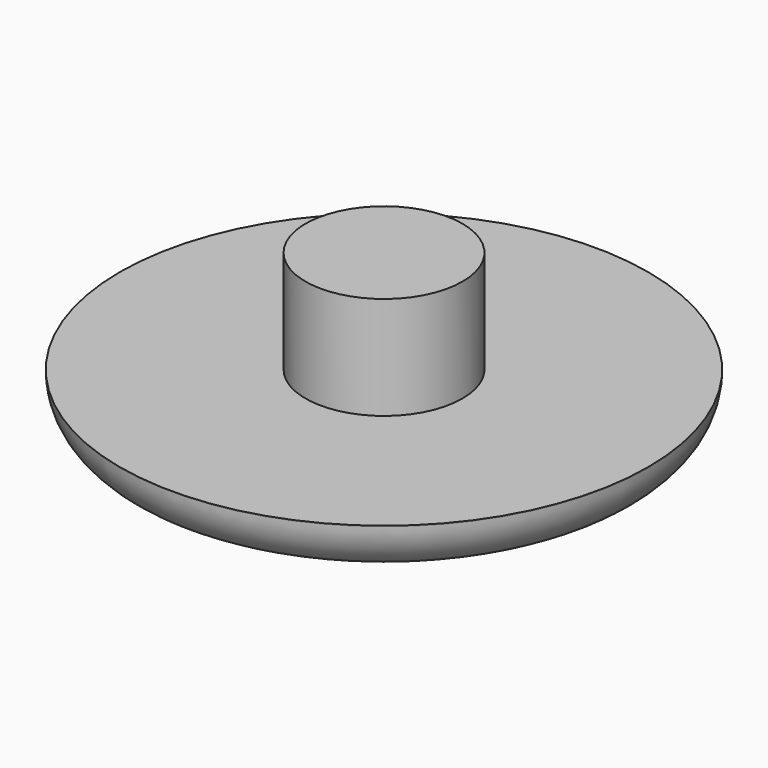
from build123d import *

# Parameters (mm, degrees)
F0_R     = 12.827
F1_DEPTH = 2.54
F2_R     = 8.89
F3_DEPTH = 0.635
F5_R     = 25.4
F7_R     = 3.81
F8_DEPTH = 5


# Not quite as in the source:
# - a fillet or chamfer that OpenCascade refuses, or shapes differently, is made with other operations: its cross-section is extruded or revolved along the edge and cut away or added


with BuildPart() as f1:
    # F0 (on Top) → F1 (new body)
    with BuildSketch(Plane.XY):
        Circle(F0_R)
    extrude(amount=-F1_DEPTH)

    # F2 (on face) → F3 (cut)
    with BuildSketch(Plane(origin=(0, 0, -2.54), x_dir=(1, 0, 0), z_dir=(0, 0, -1))):
        Circle(F2_R)
    extrude(amount=-F3_DEPTH, mode=Mode.SUBTRACT)

    # F4: fillet of radius 60.96 on 1 edges, made by hand

    # F4_s1 → F4_t2 (revolve)
    with BuildSketch(Plane.XZ):
        with BuildLine():
            ThreePointArc((8.89, -2.54), (4.5135344509, -2.0639572458), (0.1141253997, -1.905))
            Line((0.1141253997, -1.905), (8.89, -1.905))
            Line((8.89, -1.905), (8.89, -2.54))
        make_face()
    revolve(axis=Axis((0, 0, -1.905), (0, 0, -1)))

    # F5
    f5_edges = [f1.edges().sort_by_distance(p)[0] for p in [
        (-8.89, 0, -2.54),
    ]]
    fillet(f5_edges, radius=F5_R)

    # F6: fillet of radius 2.54 on 1 edges, made by hand

    # F6_s1 → F6_t2 (revolve, cut)
    with BuildSketch(Plane.XZ):
        with BuildLine():
            ThreePointArc((10.2547372433, -2.5384738057), (12.0719517601, -1.8053490766), (12.8274, 0.0026991598))
            Line((12.8274, 0.0026991598), (13.0815365685, 0.0026991598))
            ThreePointArc((13.0815365685, 0.0026991598), (13.0811365685, -1.2686504201), (13.0811365685, -2.54))
            Line((13.0811365685, -2.54), (12.827, -2.7941365685))
            ThreePointArc((12.827, -2.7941365685), (10.5675446967, -2.7941365685), (10.2516075362, -2.7925911022))
            Line((10.2516075362, -2.7925911022), (10.2547372433, -2.5384738057))
        make_face()
    revolve(axis=Axis((0, 0, -2.54), (0, 0, 1)), mode=Mode.SUBTRACT)

    # F7 (on face) → F8 (join)
    with BuildSketch(Plane.XY):
        Circle(F7_R)
    extrude(amount=F8_DEPTH)


solid = f1.part
